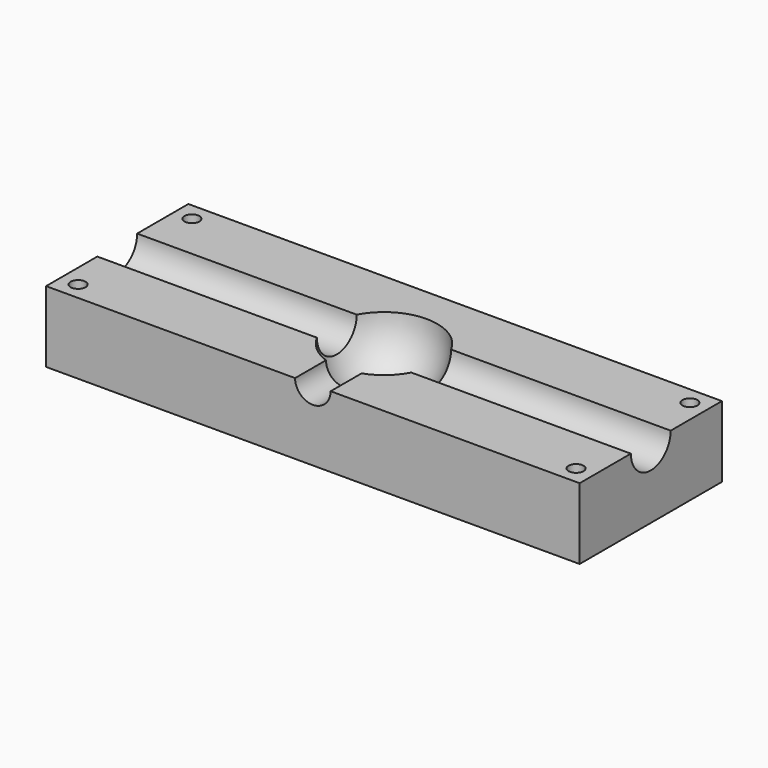
from build123d import *

# Parameters (mm, degrees)
F1_DEPTH  = 25
F5_D      = 4.2
F5_DEPTH  = 20
F5_TIP    = 1.2618073
F10_DEPTH = 50.001


with BuildPart() as f1:
    # F0 (on Front) → F1 (new body, symmetric)
    with BuildSketch(Plane.XZ):
        with BuildLine():
            ThreePointArc((0, 315), (37.7725508345, 312.7270925319), (75, 305.9411708156))
            Line((75, 305.9411708156), (75, 335))
            Line((75, 335), (0, 335))
            Line((0, 335), (0, 315))
        make_face()
        with BuildLine():
            ThreePointArc((-75, 305.9411708156), (-37.7725508345, 312.7270925319), (0, 315))
            Line((0, 315), (0, 335))
            Line((0, 335), (-75, 335))
            Line((-75, 335), (-75, 305.9411708156))
        make_face()
    extrude(amount=F1_DEPTH, both=True)

    # F2 (on face) → F3 (revolve, cut)
    with BuildSketch(Plane.XY.offset(335)):
        with BuildLine():
            Line((-13.2664991614, 7), (-75, 7))
            Line((-75, 7), (-75, 0))
            Line((-75, 0), (-15, 0))
            ThreePointArc((-15, 0), (-14.5601766373, 3.6057254872), (-13.2664991614, 7))
        make_face()
        with BuildLine():
            ThreePointArc((13.2664991614, 7), (0, 15), (-13.2664991614, 7))
            ThreePointArc((-13.2664991614, 7), (-14.5601766373, 3.6057254872), (-15, 0))
            Line((-15, 0), (-13.2664991614, 0))
            Line((-13.2664991614, 0), (13.2664991614, 0))
            Line((13.2664991614, 0), (15, 0))
            ThreePointArc((15, 0), (14.5601766373, 3.6057254872), (13.2664991614, 7))
        make_face()
        with BuildLine():
            Line((75, 7), (13.2664991614, 7))
            ThreePointArc((13.2664991614, 7), (14.5601766373, 3.6057254872), (15, 0))
            Line((15, 0), (75, 0))
            Line((75, 0), (75, 7))
        make_face()
    revolve(axis=Axis((-44.1332495807, 0, 335), (1, 0, 0)), mode=Mode.SUBTRACT)

    # F5
    with Locations(Plane.XY.offset(335)):
        with Locations((-70, 20), (-70, -20), (70, 20), (70, -20)):
            Hole(F5_D / 2, depth=F5_DEPTH)
            with Locations((0, 0, -(F5_DEPTH + F5_TIP / 2))):  # 118° drill point
                Cone(0, F5_D / 2, F5_TIP, mode=Mode.SUBTRACT)

    # F6 (on face) → F7 (revolve, cut)
    with BuildSketch(Plane.XY.offset(335)):
        with BuildLine():
            Line((0, 0), (-5, 0))
            Line((-5, 0), (-5, -14.1421356237))
            ThreePointArc((-5, -14.1421356237), (-2.5365296809, -14.7839783948), (0, -15))
            Line((0, -15), (0, 0))
        make_face()
        with BuildLine():
            ThreePointArc((0, -15), (-2.5365296809, -14.7839783948), (-5, -14.1421356237))
            Line((-5, -14.1421356237), (-5, -25))
            Line((-5, -25), (0, -25))
            Line((0, -25), (0, -15))
        make_face()
    revolve(axis=Axis((0, -12.5, 335), (0, -1, 0)), mode=Mode.SUBTRACT)

    # F9 (on face) → F10 (cut, through all)
    with BuildSketch(Plane.XZ.offset(25)):
        with BuildLine():
            ThreePointArc((0, 315), (37.7725508345, 312.7270925319), (75, 305.9411708156))
            Line((75, 305.9411708156), (75, 315))
            Line((75, 315), (0, 315))
        make_face()
        with BuildLine():
            Line((-75, 315), (-75, 305.9411708156))
            ThreePointArc((-75, 305.9411708156), (-37.7725508345, 312.7270925319), (0, 315))
            Line((0, 315), (-75, 315))
        make_face()
    extrude(amount=-F10_DEPTH, mode=Mode.SUBTRACT)


solid = f1.part
